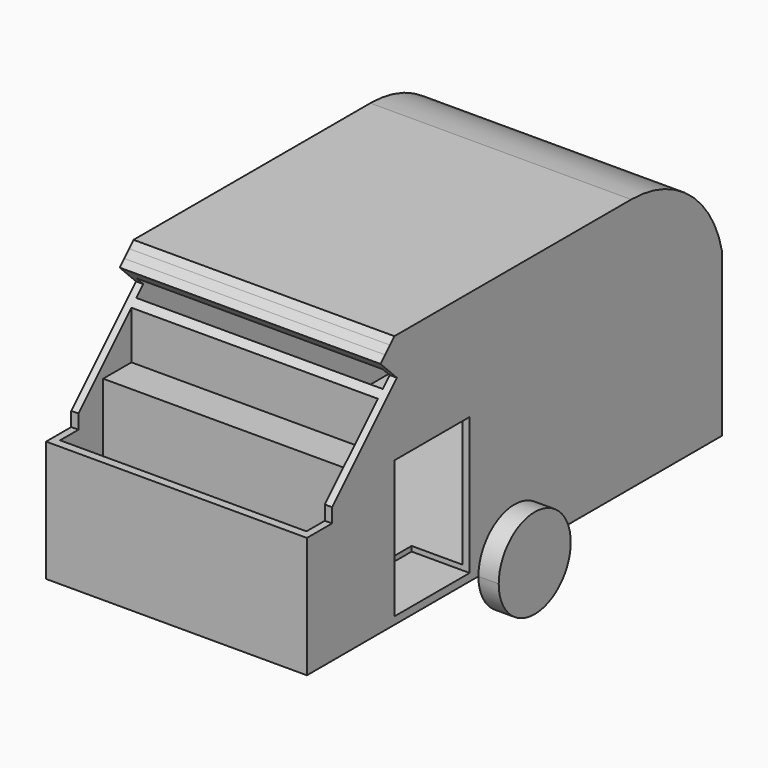
from build123d import *

# Parameters (mm, degrees)
F1_DEPTH  = 57.15
F3_DEPTH  = 5.08
F5_DEPTH  = 41.402
F7_DEPTH  = 53.975
F8_W      = 41.1952470895
F8_H      = 60.1872038096
F9_DEPTH  = 25.4
F11_DEPTH = 114.3
F12_W     = 114.3
F12_H     = 56.9759604018
F13_DEPTH = 12.7
F15_DEPTH = 114.3
F17_DEPTH = 8.89
F18_R     = 19.3940377175
F19_DEPTH = 8.89


with BuildPart() as f1:
    # F0 (on Right) → F1 (new body, symmetric)
    with BuildSketch(Plane.YZ):
        with BuildLine():
            Line((-92.7504450083, 16.9447939843), (-92.7504450083, -46.5026274323))
            Line((-92.7504450083, -46.5026274323), (134.5391124487, -46.5026274323))
            Line((134.5391124487, -46.5026274323), (134.5391124487, 24.8438697308))
            ThreePointArc((134.5391124487, 24.8438697308), (116.7467916318, 53.6046661319), (84.8513692617, 64.848870039))
            Line((84.8513692617, 64.848870039), (-44.8463708162, 64.848870039))
            Line((-44.8463708162, 64.848870039), (-92.7504450083, 16.9447939843))
        make_face()
    extrude(amount=F1_DEPTH, both=True)

    # F2 (on face) → F3 (join)
    with BuildSketch(Plane(origin=(0, 0, -46.5026274323), x_dir=(1, 0, 0), z_dir=(0, 0, -1))):
        Polygon((-28.575, -77.7167230844), (0, -134.5391124487), (28.575, -77.7167230844), (57.15, -20.8943337202), (-57.15, -20.8943337202), align=None)
        Polygon((28.575, -77.7167230844), (0, -134.5391124487), (8.5433015109, -134.5391124487), align=None)
        Polygon((-8.5433015109, -134.5391124487), (0, -134.5391124487), (-28.575, -77.7167230844), align=None)
        Polygon((8.5433015109, -134.5391124487), (0, -134.5391124487), (-8.5433015109, -134.5391124487), (0, -158.7732434273), align=None)
    extrude(amount=-F3_DEPTH)

    # F4 (on face) → F5 (cut)
    with BuildSketch(Plane(origin=(0, 0, -46.5026274323), x_dir=(1, 0, 0), z_dir=(0, 0, -1))):
        Polygon((-4.6747997403, -134.5391124487), (0, -146.656177938), (4.2716507554, -134.5391124487), align=None)
    extrude(amount=-F5_DEPTH, mode=Mode.SUBTRACT)

    # F6 (on Right) → F7 (cut, symmetric)
    with BuildSketch(Plane.YZ):
        with BuildLine():
            Line((-89.0294536948, 15.1805384085), (-89.0294536948, -41.0569272935))
            Line((-89.0294536948, -41.0569272935), (130.7652890682, -41.0569272935))
            Line((130.7652890682, -41.0569272935), (130.7652890682, 25.959385559))
            ThreePointArc((130.7652890682, 25.959385559), (115.7413511895, 50.5424798047), (88.5871946812, 60.1705126464))
            Line((88.5871946812, 60.1705126464), (-44.0394952893, 60.1705126464))
            Line((-44.0394952893, 60.1705126464), (-89.0294536948, 15.1805384085))
        make_face()
    extrude(amount=F7_DEPTH, both=True, mode=Mode.SUBTRACT)

    # F8 (on face) → F9 (cut, symmetric)
    with BuildSketch(Plane.YZ.offset(57.15)):
        with Locations((-24.2487472715, -13.1488079205)):
            Rectangle(F8_W, F8_H)
    extrude(amount=F9_DEPTH, both=True, mode=Mode.SUBTRACT)

    # F10 (on face) → F11 (join)
    with BuildSketch(Plane.YZ.offset(57.15)):
        Polygon((-92.7504450083, -11.7301335558), (-92.7504450083, -14.778916724), (-47.2835078835, -14.778916724), (-47.2835078835, -11.7301335558), (-63.0396455526, -11.7301335558), (-63.0396455526, 16.9447939843), (-47.2835078835, 16.9447939843), (-47.2835078835, 62.4117328769), (-49.9636399546, 59.7316007017), (-49.9636399546, 20.691152662), (-65.4636770487, 20.691152662), (-65.4636770487, -11.7301335558), align=None)
    extrude(amount=-F11_DEPTH)

    # F12 (on face) → F13 (cut)
    with BuildSketch(Plane(origin=(0, -54.8476212995, 54.8476191669), x_dir=(1, 0, 0), z_dir=(0, -0.7071067949, 0.7071067674))):
        with Locations((0, -25.1147081824)):
            Rectangle(F12_W, F12_H)
    extrude(amount=-F13_DEPTH, mode=Mode.SUBTRACT)

    # F14 (on face) → F15 (cut)
    with BuildSketch(Plane.YZ.offset(57.15)):
        Polygon((-92.7504450083, 16.9447939843), (-92.7504450083, 6.4976271242), (-78.9771229029, 6.4976271242), (-78.9771229029, 12.7576040339), (-83.7701887126, 7.9645380378), align=None)
    extrude(amount=-F15_DEPTH, mode=Mode.SUBTRACT)

    # F16 (on face) → F17 (join)
    with BuildSketch(Plane.YZ.offset(57.15)):
        with BuildLine():
            Line((20.8943337202, -46.5026274323), (40.6107781849, -46.5026274323))
            ThreePointArc((40.6107781849, -46.5026274323), (20.8943337202, -26.7861829676), (1.1778892555, -46.5026274323))
            Line((1.1778892555, -46.5026274323), (20.8943337202, -46.5026274323))
        make_face()
        with BuildLine():
            ThreePointArc((1.1778892555, -46.5026274323), (20.8943337202, -66.2190718971), (40.6107781849, -46.5026274323))
            Line((40.6107781849, -46.5026274323), (20.8943337202, -46.5026274323))
            Line((20.8943337202, -46.5026274323), (1.1778892555, -46.5026274323))
        make_face()
    extrude(amount=F17_DEPTH)

    # F18 (on face) → F19 (join)
    with BuildSketch(Plane(origin=(-57.15, 0, 0), x_dir=(0, -1, 0), z_dir=(-1, 0, 0))):
        with Locations((-20.8943337202, -46.5026274323)):
            Circle(F18_R)
    extrude(amount=F19_DEPTH)


solid = f1.part
